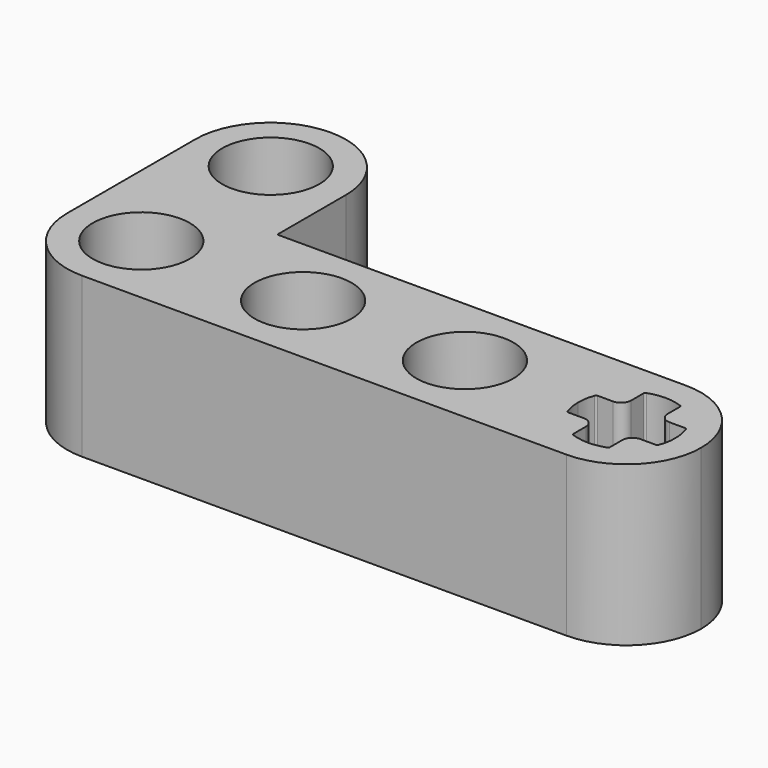
from build123d import *

# Parameters (mm, degrees)
F0_R        = 2.4
F0_W        = 7.4481110471
F0_H        = 7.95
F1_DEPTH    = 7.88
F2_T1_DEPTH = 26.405


# Not quite as in the source:
# - a fillet or chamfer that OpenCascade refuses, or shapes differently, is made with other operations: its cross-section is extruded or revolved along the edge and cut away or added


with BuildPart() as f1:
    # F0 (on Top) → F1 (new body)
    with BuildSketch(Plane.XY):
        Polygon((-17.0395083171, 1.6058013724), (-28.7195083171, 1.6058013724), (-40.95139727, 1.6058013724), (-48.3995083171, 1.6058013724), (-48.3995083171, -5.7841986276), (-31.3221290569, -5.7841986276), (-17.0395083171, -5.7841986276), align=None)
        with Locations((-44.7195083171, -2.0891986276)):
            Circle(F0_R, mode=Mode.SUBTRACT)
        with Locations((-36.7195083171, -2.0891986276)):
            Circle(F0_R, mode=Mode.SUBTRACT)
        with BuildLine():
            ThreePointArc((-28.7195083171, -4.4891986276), (-31.1195083171, -2.0891986276), (-28.7195083171, 0.3108013724))
            ThreePointArc((-28.7195083171, 0.3108013724), (-26.3195083171, -2.0891986276), (-28.7195083171, -4.4891986276))
        make_face(mode=Mode.SUBTRACT)
        with BuildLine():
            ThreePointArc((-22.1195083171, -1.1891986276), (-21.7659549265, -1.0427520182), (-21.6195083171, -0.6891986276))
            Line((-21.6195083171, -0.6891986276), (-21.6195083171, 0.0671872376))
            ThreePointArc((-21.6195083171, 0.0671872376), (-21.601600524, 0.1242912617), (-21.5542909257, 0.1609431448))
            ThreePointArc((-21.5542909257, 0.1609431448), (-20.7195083171, 0.3108013724), (-19.8847257084, 0.1609431448))
            ThreePointArc((-19.8847257084, 0.1609431448), (-19.8374161101, 0.1242912617), (-19.8195083171, 0.0671872376))
            Line((-19.8195083171, 0.0671872376), (-19.8195083171, -0.6891986276))
            ThreePointArc((-19.8195083171, -0.6891986276), (-19.6730617076, -1.0427520182), (-19.3195083171, -1.1891986276))
            Line((-19.3195083171, -1.1891986276), (-18.5631224518, -1.1891986276))
            ThreePointArc((-18.5631224518, -1.1891986276), (-18.5060184277, -1.2071064207), (-18.4693665446, -1.2544160189))
            ThreePointArc((-18.4693665446, -1.2544160189), (-18.3572699449, -1.6651351029), (-18.3195083171, -2.0891986276))
            ThreePointArc((-18.3195083171, -2.0891986276), (-18.3572699449, -2.5132621524), (-18.4693665446, -2.9239812363))
            ThreePointArc((-18.4693665446, -2.9239812363), (-18.5060184277, -2.9712908345), (-18.5631224518, -2.9891986276))
            Line((-18.5631224518, -2.9891986276), (-19.3195083171, -2.9891986276))
            ThreePointArc((-19.3195083171, -2.9891986276), (-19.6730617076, -3.135645237), (-19.8195083171, -3.4891986276))
            Line((-19.8195083171, -3.4891986276), (-19.8195083171, -4.2455844929))
            ThreePointArc((-19.8195083171, -4.2455844929), (-19.8374161101, -4.302688517), (-19.8847257084, -4.3393404001))
            ThreePointArc((-19.8847257084, -4.3393404001), (-20.7195083171, -4.4891986276), (-21.5542909257, -4.3393404001))
            ThreePointArc((-21.5542909257, -4.3393404001), (-21.601600524, -4.302688517), (-21.6195083171, -4.2455844929))
            Line((-21.6195083171, -4.2455844929), (-21.6195083171, -3.4891986276))
            ThreePointArc((-21.6195083171, -3.4891986276), (-21.7659549265, -3.135645237), (-22.1195083171, -2.9891986276))
            Line((-22.1195083171, -2.9891986276), (-22.8758941823, -2.9891986276))
            ThreePointArc((-22.8758941823, -2.9891986276), (-22.9329982064, -2.9712908345), (-22.9696500895, -2.9239812363))
            ThreePointArc((-22.9696500895, -2.9239812363), (-23.0817466892, -2.5132621524), (-23.1195083171, -2.0891986276))
            ThreePointArc((-23.1195083171, -2.0891986276), (-23.0817466892, -1.6651351029), (-22.9696500895, -1.2544160189))
            ThreePointArc((-22.9696500895, -1.2544160189), (-22.9329982064, -1.2071064207), (-22.8758941823, -1.1891986276))
            Line((-22.8758941823, -1.1891986276), (-22.1195083171, -1.1891986276))
        make_face(mode=Mode.SUBTRACT)
        with Locations((-44.6754527935, 5.5808013724)):
            Rectangle(F0_W, F0_H)
        with Locations((-44.7195083171, 5.9108013724)):
            Circle(F0_R, mode=Mode.SUBTRACT)
    extrude(amount=F1_DEPTH)

    # F2: fillet of radius 3.705 on 5 edges, made by hand

    # F2_s2 → F2_t1 (cut)
    with BuildSketch(Plane.XY.offset(-9.2625)):
        with BuildLine():
            ThreePointArc((-44.6945083171, 9.5558013724), (-47.3143389413, 8.4706319967), (-48.3995083171, 5.8508013724))
            Line((-48.3995083171, 5.8508013724), (-48.3995083171, 9.5558013724))
            Line((-48.3995083171, 9.5558013724), (-44.6945083171, 9.5558013724))
        make_face()
        with BuildLine():
            ThreePointArc((-40.95139727, 5.8508013724), (-42.0365666457, 8.4706319967), (-44.65639727, 9.5558013724))
            Line((-44.65639727, 9.5558013724), (-40.95139727, 9.5558013724))
            Line((-40.95139727, 9.5558013724), (-40.95139727, 5.8508013724))
        make_face()
        with BuildLine():
            ThreePointArc((-48.3995083171, -2.0791986276), (-47.3143389413, -4.6990292519), (-44.6945083171, -5.7841986276))
            Line((-44.6945083171, -5.7841986276), (-48.3995083171, -5.7841986276))
            Line((-48.3995083171, -5.7841986276), (-48.3995083171, -2.0791986276))
        make_face()
        with BuildLine():
            ThreePointArc((-17.0395083171, -2.0991986276), (-18.1246776928, 0.5206319967), (-20.7445083171, 1.6058013724))
            Line((-20.7445083171, 1.6058013724), (-17.0395083171, 1.6058013724))
            Line((-17.0395083171, 1.6058013724), (-17.0395083171, -2.0991986276))
        make_face()
        with BuildLine():
            ThreePointArc((-17.0395083171, -2.0791986276), (-18.1246776928, -4.6990292519), (-20.7445083171, -5.7841986276))
            Line((-20.7445083171, -5.7841986276), (-17.0395083171, -5.7841986276))
            Line((-17.0395083171, -5.7841986276), (-17.0395083171, -2.0791986276))
        make_face()
    extrude(amount=F2_T1_DEPTH, mode=Mode.SUBTRACT)


solid = f1.part
